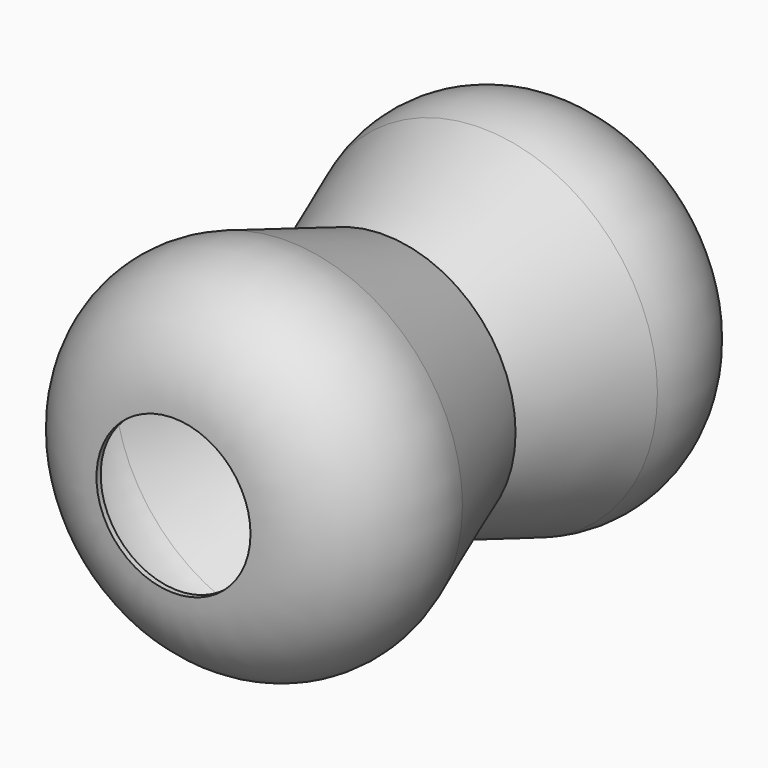
from build123d import *

# Parameters (mm, degrees)
F0_R     = 63.5
F1_DEPTH = 127
F1_TAPER = -20
F2_R     = 50.8
F3_T     = -2.54


# Not quite as in the source:
# - a shell that OpenCascade refuses in one call is made with other operations: the cavity is built on its own and cut out


with BuildPart() as f1:
    # F0 (on Front) → F1 (new body, symmetric)
    with BuildSketch(Plane.XZ):
        Circle(F0_R)
    extrude(amount=F1_DEPTH, both=True, taper=F1_TAPER)

    # F2
    f2_edges = [f1.edges().sort_by_distance(p)[0] for p in [
        (-109.72422, -127, 0),
        (-109.72422, 127, 0),
    ]]
    fillet(f2_edges, radius=F2_R)

    # F3: a shell. OpenCascade refuses it in one call, so the cavity is built on its own and cut out:
    # the body offset inwards by the wall thickness, plus a prism from it out through each open face.
    f3_core = offset(f1.part, amount=F3_T, kind=Kind.INTERSECTION, mode=Mode.PRIVATE)
    f3_exits = [f3_core.faces().sort_by_distance(p)[0] for p in [
        (0, -124.46, 0),
    ]]
    add(f3_core, mode=Mode.SUBTRACT)
    extrude(f3_exits, amount=-F3_T, mode=Mode.SUBTRACT)


solid = f1.part
